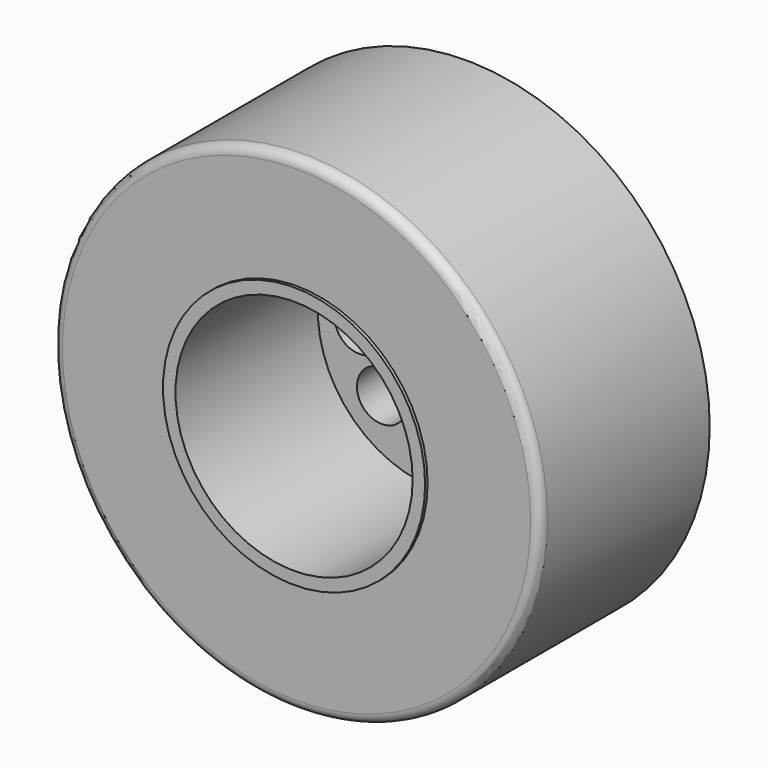
from build123d import *
from build123d import SkipClean  # not in build123d's __all__

# Parameters (mm, degrees)
F0_R      = 19.5
F1_DEPTH  = 17
F2_R      = 9.5
F3_DEPTH  = 14
F4_R      = 18.5
F4_R_2    = 10.5
F5_DEPTH  = 16
F6_R      = 2
F7_DEPTH  = 25
F8_R      = 3.5
F9_DEPTH  = 4
F10_R     = 2
F11_DEPTH = 138.7
F12_R     = 4
F12_R_2   = 2
F13_DEPTH = 1
F14_R     = 2.5
F14_R_2   = 2
F15_DEPTH = 0.75
F16_R     = 0.5
F17_DEPTH = 0.5
F19_R     = 0.75
F18_R     = 10.5
F18_R_2   = 9.5
F20_DEPTH = 0.25


# Not quite as in the source:
# - after a boolean that leaves OpenCascade's solid faulty, fix() repairs it


with BuildPart() as f1:
    # F0 (on Front) → F1 (new body)
    with BuildSketch(Plane.XZ):
        Circle(F0_R)
    extrude(amount=F1_DEPTH)

    # F2 (on face) → F3 (cut)
    with BuildSketch(Plane.XZ.offset(17)):
        Circle(F2_R)
    extrude(amount=-F3_DEPTH, mode=Mode.SUBTRACT)

    # F4 (on face) → F5 (cut)
    with BuildSketch(Plane(origin=(0, 0, 0), x_dir=(-1, 0, 0), z_dir=(0, 1, 0))):
        Circle(F4_R)
        Circle(F4_R_2, mode=Mode.SUBTRACT)
    extrude(amount=-F5_DEPTH, mode=Mode.SUBTRACT)

    # F6 (on face) → F7 (cut)
    with BuildSketch(Plane.XZ.offset(3)):
        with Locations((0, 6.1688632704)):
            Circle(F6_R)
        with Locations((-4.3620450507, 4.3620450507)):
            Circle(F6_R)
        with Locations((-6.1688632704, 0)):
            Circle(F6_R)
        with Locations((-4.3620450507, -4.3620450507)):
            Circle(F6_R)
        with Locations((0, -6.1688632704)):
            Circle(F6_R)
        with Locations((4.3620450507, -4.3620450507)):
            Circle(F6_R)
        with Locations((6.1688632704, 0)):
            Circle(F6_R)
        with Locations((4.3620450507, 4.3620450507)):
            Circle(F6_R)
    extrude(amount=-F7_DEPTH, mode=Mode.SUBTRACT)

    # F8 (on face) → F9 (join)
    with BuildSketch(Plane(origin=(0, 0, 0), x_dir=(-1, 0, 0), z_dir=(0, 1, 0))):
        Circle(F8_R)
    extrude(amount=F9_DEPTH)

    # F10 (on face) → F11 (cut)
    with BuildSketch(Plane(origin=(0, 4, 0), x_dir=(-1, 0, 0), z_dir=(0, 1, 0))):
        Circle(F10_R)
    extrude(amount=-F11_DEPTH, mode=Mode.SUBTRACT)

    # F12 (on face) → F13 (join)
    with BuildSketch(Plane.XZ.offset(3)):
        with Locations((0.0866679911, 0.0506265242)):
            Circle(F12_R)
        Circle(F12_R_2, mode=Mode.SUBTRACT)
    with SkipClean():  # cleaning this boolean's faces spoils the solid; the shape is the same uncleaned
        extrude(amount=F13_DEPTH)

    # F14 (on face) → F15 (join)
    with BuildSketch(Plane.XZ.offset(4)):
        Circle(F14_R)
        Circle(F14_R_2, mode=Mode.SUBTRACT)
    extrude(amount=F15_DEPTH)

    add(f1.part.fix(), mode=Mode.REPLACE)

    # F16 (on face) → F17 (join)
    with BuildSketch(Plane.XZ.offset(4)):
        with Locations((0, 3.2079922967)):
            Circle(F16_R)
        with Locations((-1.8856105614, 2.5953202858)):
            Circle(F16_R)
        with Locations((-3.050981978, 0.9913241375)):
            Circle(F16_R)
        with Locations((-3.050981978, -0.9913241375)):
            Circle(F16_R)
        with Locations((-1.8856105614, -2.5953202858)):
            Circle(F16_R)
        with Locations((0, -3.2079922967)):
            Circle(F16_R)
        with Locations((1.8856105614, -2.5953202858)):
            Circle(F16_R)
        with Locations((3.050981978, -0.9913241375)):
            Circle(F16_R)
        with Locations((3.050981978, 0.9913241375)):
            Circle(F16_R)
        with Locations((1.8856105614, 2.5953202858)):
            Circle(F16_R)
    extrude(amount=F17_DEPTH)

    # F19
    f19_edges = [f1.edges().sort_by_distance(p)[0] for p in [
        (-19.5, -17, 0),
    ]]
    fillet(f19_edges, radius=F19_R)

    # F18 (on face) → F20 (join)
    with BuildSketch(Plane.XZ.offset(17)):
        Circle(F18_R)
        Circle(F18_R_2, mode=Mode.SUBTRACT)
    extrude(amount=F20_DEPTH)


solid = f1.part
